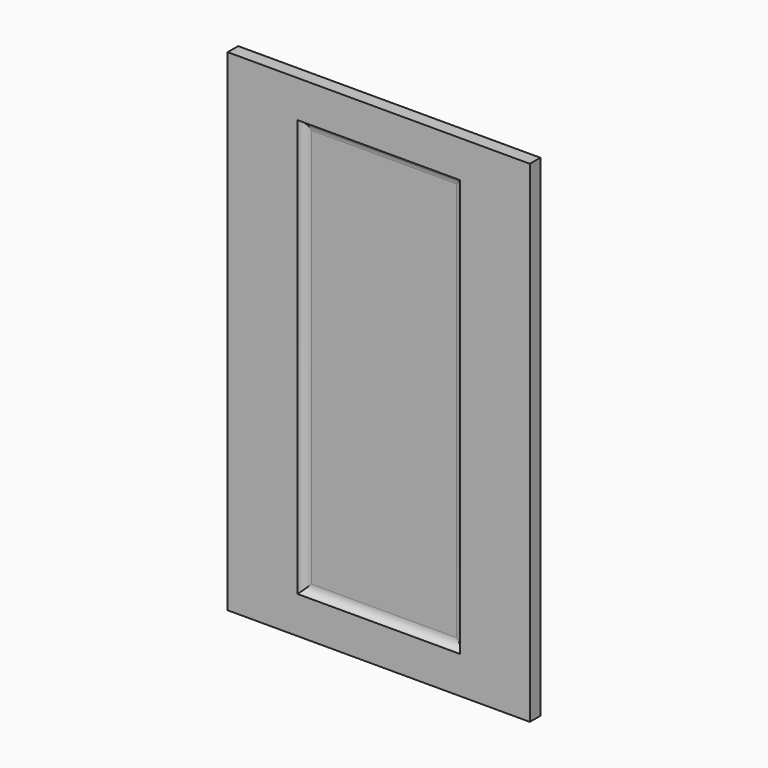
from build123d import *

# Parameters (mm, degrees)
F0_W        = 292.1
F0_H        = 474.98
F1_DEPTH    = 12.7
F2_W        = 157.1649909019
F2_H        = 403.2308459282
F3_DEPTH    = 6.35
F4_T1_DEPTH = 445.8279408996
F4_T3_DEPTH = 199.7620858733


# Not quite as in the source:
# - a fillet or chamfer that OpenCascade refuses, or shapes differently, is made with other operations: its cross-section is extruded or revolved along the edge and cut away or added


with BuildPart() as f1:
    # F0 (on Front) → F1 (new body)
    with BuildSketch(Plane.XZ):
        Rectangle(F0_W, F0_H)
    extrude(amount=F1_DEPTH)

    # F2 (on face) → F3 (cut)
    with BuildSketch(Plane.XZ.offset(12.7)):
        Rectangle(F2_W, F2_H)
    extrude(amount=-F3_DEPTH, mode=Mode.SUBTRACT)

    # F4: fillet of radius 8.89 on 4 edges, made by hand

    # F4_s2 → F4_t1 (join)
    with BuildSketch(Plane.XY.offset(-222.9139704498)):
        with BuildLine():
            ThreePointArc((78.582495451, -12.7), (75.3758676252, -8.1121426782), (70.0630764567, -6.35))
            Line((70.0630764567, -6.35), (78.582495451, -6.35))
            Line((78.582495451, -6.35), (78.582495451, -12.7))
        make_face()
        with BuildLine():
            ThreePointArc((-78.582495451, -12.7), (-75.3758676252, -8.1121426782), (-70.0630764567, -6.35))
            Line((-70.0630764567, -6.35), (-78.582495451, -6.35))
            Line((-78.582495451, -6.35), (-78.582495451, -12.7))
        make_face()
    extrude(amount=F4_T1_DEPTH)

    # F4_s4 → F4_t3 (join)
    with BuildSketch(Plane.YZ.offset(-99.8810429367)):
        with BuildLine():
            ThreePointArc((-12.7, 201.6154229641), (-8.1121426782, 198.4087951383), (-6.35, 193.0960039698))
            Line((-6.35, 193.0960039698), (-6.35, 201.6154229641))
            Line((-6.35, 201.6154229641), (-12.7, 201.6154229641))
        make_face()
        with BuildLine():
            ThreePointArc((-12.7, -201.6154229641), (-8.1121426782, -198.4087951383), (-6.35, -193.0960039698))
            Line((-6.35, -193.0960039698), (-6.35, -201.6154229641))
            Line((-6.35, -201.6154229641), (-12.7, -201.6154229641))
        make_face()
    extrude(amount=F4_T3_DEPTH)


solid = f1.part
